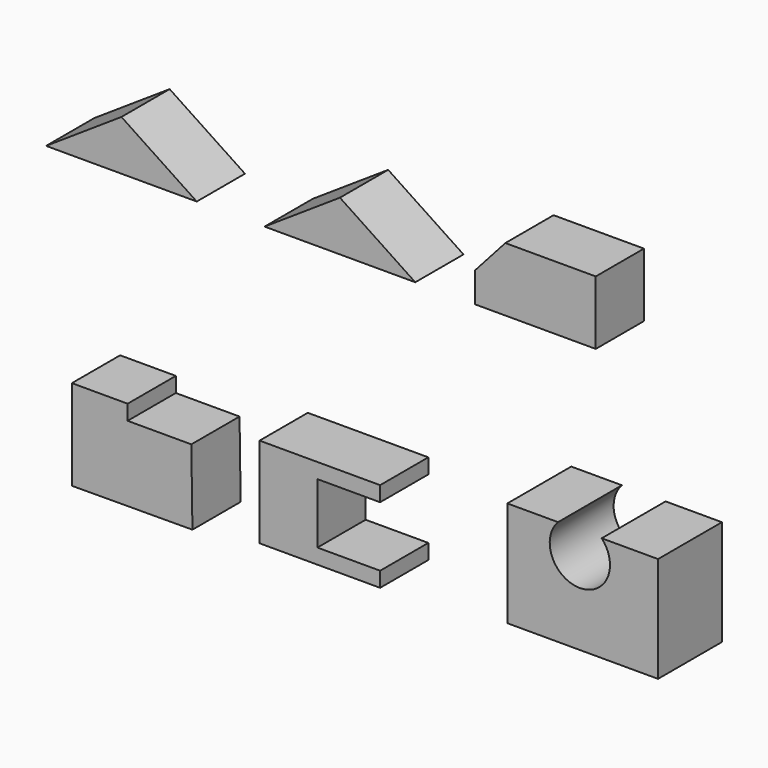
from build123d import *

# Parameters (mm, degrees)
F1_DEPTH  = 101.6
F3_DEPTH  = 101.6
F4_W      = 101.6
F4_H      = 50.8
F5_DEPTH  = 101.6
F7_DEPTH  = 101.6
F9_DEPTH  = 101.6
F11_DEPTH = 101.6
F13_DEPTH = 134.62


with BuildPart() as f1:
    # F0 (on Front) → F1 (new body)
    with BuildSketch(Plane.XZ):
        Polygon((0, 84.242269675), (-127, 0), (127, 0), align=None)
    extrude(amount=F1_DEPTH)

    # F8 (on Front) → F9 (cut)
    with BuildSketch(Plane.XZ):
        Polygon((352.6244014331, -321.0040116787), (352.6244014331, -473.4040116787), (555.8244014331, -473.4040116787), (555.8244014331, -448.0040116787), (454.2244014331, -448.0040116787), (454.2244014331, -346.4040116787), (555.8244014331, -346.4040116787), (555.8244014331, -321.0040116787), align=None)
    extrude(amount=-F9_DEPTH, mode=Mode.SUBTRACT)


with BuildPart() as f3:
    # F2 (on Front) → F3 (new body)
    with BuildSketch(Plane.XZ):
        Polygon((368.3589263118, 84.242269675), (241.3589263118, 0), (495.3589263118, 0), align=None)
    extrude(amount=F3_DEPTH)


with BuildPart() as f5:
    # F4 (on Front) → F5 (new body)
    with BuildSketch(Plane.XZ):
        Polygon((596.3775763313, 50.8), (596.3775763313, 0), (697.9775763313, 0), (697.9775763313, 50.8), (647.1775763313, 107.5961266285), align=None)
        Polygon((799.5775763313, 107.5961266285), (647.1775763313, 107.5961266285), (697.9775763313, 50.8), (799.5775763313, 50.8), align=None)
        with Locations((748.7775763313, 25.4)):
            Rectangle(F4_W, F4_H)
    extrude(amount=F5_DEPTH)


with BuildPart() as f7:
    # F6 (on Front) → F7 (new body)
    with BuildSketch(Plane.XZ):
        Polygon((10.4466769844, -337.9140185932), (-83.4813854448, -337.9140185932), (-83.4813854448, -490.3140185932), (119.7163752071, -489.3600447649), (117.838434875, -363.3140185932), (10.4466769844, -363.3140185932), align=None)
    extrude(amount=F7_DEPTH)


with BuildPart() as f11:
    # F10 (on Front) → F11 (new body)
    with BuildSketch(Plane.XZ):
        Polygon((232.8759941101, -320.3524975159), (232.8759941101, -472.7524975159), (436.0759941101, -472.7524975159), (436.0759941101, -447.3524975159), (330.4120034046, -447.3524975159), (330.4120034046, -345.7524975159), (436.0759941101, -345.7524975159), (436.0759941101, -320.3524975159), align=None)
    extrude(amount=F11_DEPTH)


with BuildPart() as f13:
    # F12 (on Front) → F13 (new body)
    with BuildSketch(Plane.XZ):
        with BuildLine():
            Line((676.9858937263, -255.6922041467), (676.9858937263, -433.4922041467))
            Line((676.9858937263, -433.4922041467), (930.9858937263, -433.4922041467))
            Line((930.9858937263, -433.4922041467), (930.9858937263, -255.6922041467))
            Line((930.9858937263, -255.6922041467), (836.0171303992, -255.6922041467))
            ThreePointArc((836.0171303992, -255.6922041467), (799.2145717144, -341.5095095006), (762.4120130296, -255.6922041467))
            Line((762.4120130296, -255.6922041467), (676.9858937263, -255.6922041467))
        make_face()
    extrude(amount=F13_DEPTH)


solid = Compound([f1.part, f3.part, f5.part, f7.part, f11.part, f13.part])
